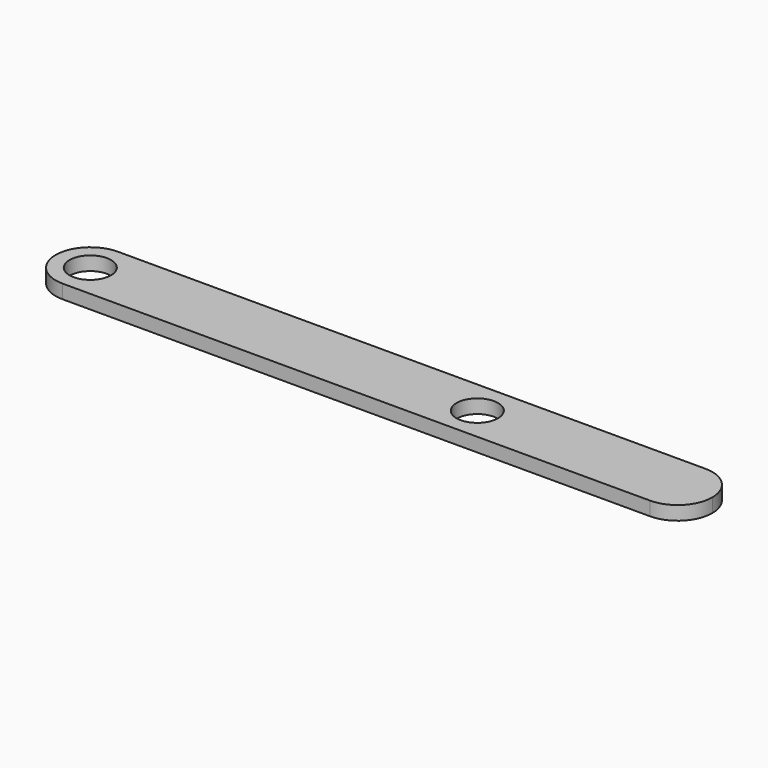
from build123d import *

# Parameters (mm, degrees)
F0_W     = 190
F0_H     = 20
F1_DEPTH = 4
F2_R     = 6
F3_DEPTH = 4.001
F4_R     = 9.99999


# Not quite as in the source:
# - a fillet or chamfer is up to 0.001 mm smaller than in the source, because OpenCascade refuses the exact size


with BuildPart() as f1:
    # F0 (on Top) → F1 (new body)
    with BuildSketch(Plane.XY):
        Rectangle(F0_W, F0_H)
    extrude(amount=F1_DEPTH)

    # F2 (on face) → F3 (cut, through all)
    with BuildSketch(Plane.XY.offset(4)):
        with Locations((-85, 0)):
            Circle(F2_R)
        with Locations((27, 0)):
            Circle(F2_R)
    extrude(amount=-F3_DEPTH, mode=Mode.SUBTRACT)

    # F4 (radius 10 in the source; OpenCascade refuses exactly that, so slightly less here)
    f4_edges = [f1.edges().sort_by_distance(p)[0] for p in [
        (-95, -10, 2),
        (-95, 10, 2),
        (95, 10, 2),
        (95, -10, 2),
    ]]
    fillet(f4_edges, radius=F4_R)


solid = f1.part
